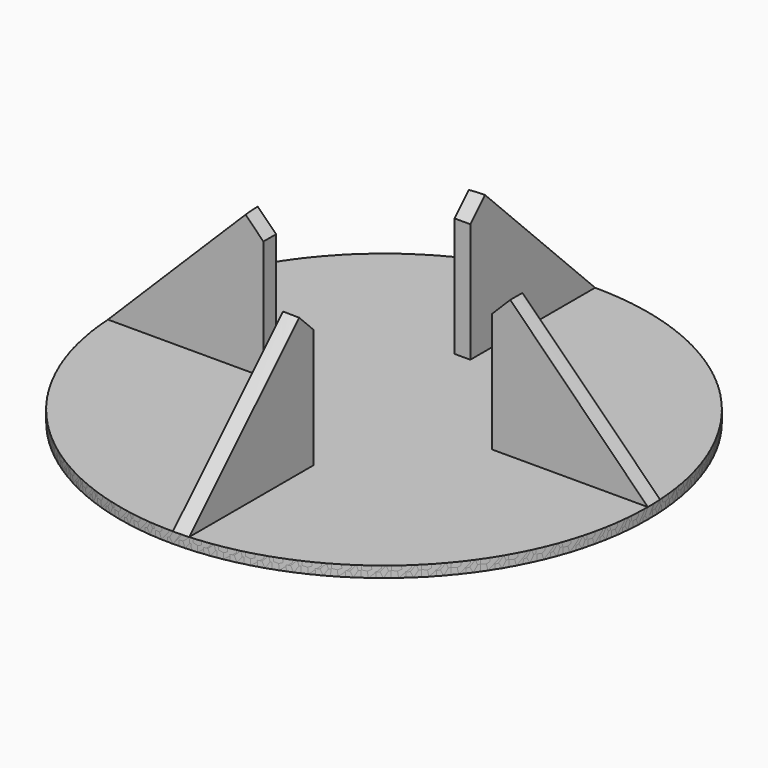
from build123d import *

# Parameters (mm, degrees)
F0_R        = 73.0403665197
F1_DEPTH    = 3.048
F3_DEPTH    = 38.1
F4_T2_ANGLE = 157.1636036311
F5_T1_DEPTH = 30.5146571208
F7_COUNT    = 4
F7_ANGLE    = 270


# Not quite as in the source:
# - a fillet or chamfer that OpenCascade refuses, or shapes differently, is made with other operations: its cross-section is extruded or revolved along the edge and cut away or added


with BuildPart() as f1:
    # F0 (on Top) → F1 (new body)
    with BuildSketch(Plane.XY):
        Circle(F0_R)
    extrude(amount=F1_DEPTH)

    # F2 (on face) → F3 (join)
    with BuildSketch(Plane.XY.offset(3.048)):
        with BuildLine():
            Line((29.8703238368, 0), (73.0403665197, 0))
            ThreePointArc((73.0403665197, 0), (73.0074021085, 2.194169249), (72.9085386299, 4.3863579631))
            Line((72.9085386299, 4.3863579631), (29.8703238368, 4.3863579631))
            Line((29.8703238368, 4.3863579631), (29.8703238368, 0))
        make_face()
    extrude(amount=F3_DEPTH)

    # F4: chamfer of 38.1 on 1 edges, made by hand

    # F4_s1 → F4_t2 (revolve, cut)
    with BuildSketch(Plane(origin=(0, 0, 0), x_dir=(0, 0, 1), z_dir=(-0.9738188817, -0.227325286, 0))):
        Polygon((3.048, -73.0403665197), (41.148, -34.9403665197), (41.148, -73.0403665197), align=None)
    revolve(axis=Axis((0, 0, 41.148), (0, 0, 1)), revolution_arc=F4_T2_ANGLE, mode=Mode.SUBTRACT)

    # F5: chamfer of 5.08 on 1 edges, made by hand

    # F5_s2 → F5_t1 (cut)
    with BuildSketch(Plane.XZ.offset(-17.450507542)):
        Polygon((34.9503238368, 41.148), (29.8703238368, 36.068), (29.8703238368, 41.148), align=None)
    extrude(amount=F5_T1_DEPTH, mode=Mode.SUBTRACT)


with BuildPart() as f7_1:
    # F7: instance of F1
    add(f1.part.rotate(Axis((0, 0, 24.7502550483), (0, 0, 1)), 1 * F7_ANGLE / (F7_COUNT - 1)))


with BuildPart() as f7_2:
    # F7: instance of F1
    add(f1.part.rotate(Axis((0, 0, 24.7502550483), (0, 0, 1)), 2 * F7_ANGLE / (F7_COUNT - 1)))


with BuildPart() as f7_3:
    # F7: instance of F1
    add(f1.part.rotate(Axis((0, 0, 24.7502550483), (0, 0, 1)), 3 * F7_ANGLE / (F7_COUNT - 1)))


solid = Compound([f1.part, f7_1.part, f7_2.part, f7_3.part])
